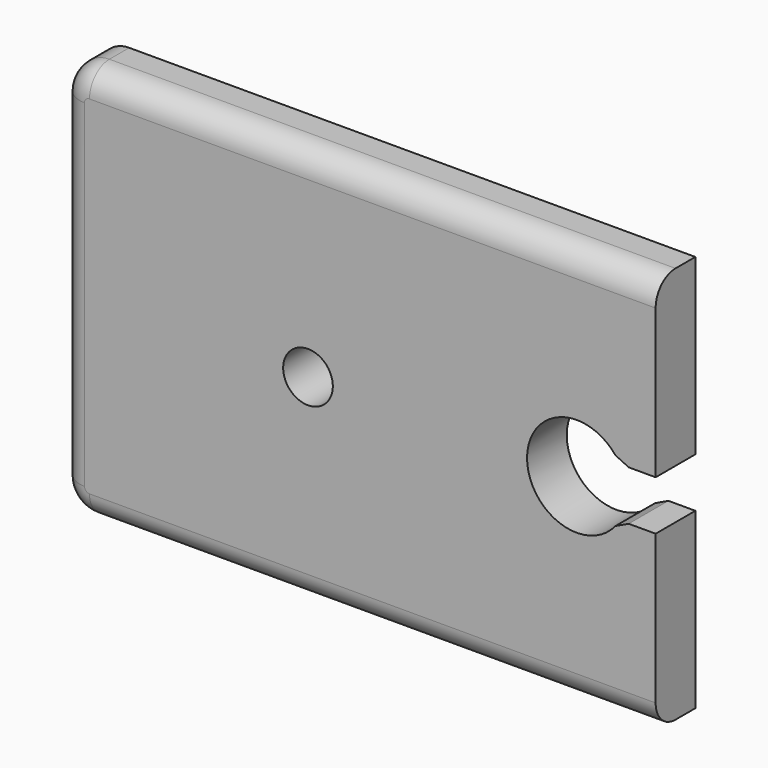
from build123d import *

# Parameters (mm, degrees)
F0_R        = 5
F1_DEPTH    = 10
F2_DEPTH    = 23.2
F3_R        = 6
F4_T1_DEPTH = 19.4160695157
F5_R        = 5


# Not quite as in the source:
# - a fillet or chamfer that OpenCascade refuses, or shapes differently, is made with other operations: its cross-section is extruded or revolved along the edge and cut away or added


with BuildPart() as f1:
    # F0 (on Front) → F1 (new body)
    with BuildSketch(Plane.XZ):
        with BuildLine():
            Line((53.1680434942, 40), (-66.8319565058, 40))
            Line((-66.8319565058, 40), (-66.8319565058, -40))
            Line((-66.8319565058, -40), (53.1680434942, -40))
            Line((53.1680434942, -40), (53.1680434942, -5))
            Line((53.1680434942, -5), (47.2735762596, -5))
            Line((47.2735762596, -5), (45.9338302975, -5))
            ThreePointArc((45.9338302975, -5), (27.2735762596, 0), (45.9338302975, 5))
            Line((45.9338302975, 5), (47.2735762596, 5))
            Line((47.2735762596, 5), (53.1680434942, 5))
            Line((53.1680434942, 5), (53.1680434942, 40))
        make_face()
        with Locations((-16.8319565058, 0)):
            Circle(F0_R, mode=Mode.SUBTRACT)
    extrude(amount=F1_DEPTH)

    # F0 (on Front) → F2 (cut)
    with BuildSketch(Plane.XZ):
        with Locations((-16.8319565058, 0)):
            Circle(F0_R)
    extrude(amount=-F2_DEPTH, mode=Mode.SUBTRACT)

    # F3
    f3_edges = [f1.edges().sort_by_distance(p)[0] for p in [
        (-66.831957, -5, -40),
        (-66.831957, -5, 40),
    ]]
    fillet(f3_edges, radius=F3_R)

    # F4: chamfer of 2 on 2 edges, made by hand

    # F4_s2 → F4_t1 (cut)
    with BuildSketch(Plane.XZ.offset(-4.7080347579)):
        with BuildLine():
            Line((44.9783315762, -6.3208937548), (47.8167286643, -4.9655276174))
            Line((47.8167286643, -4.9655276174), (47.8167286643, -4.9255276174))
            ThreePointArc((47.8167286643, -4.9255276174), (46.8752794809, -4.96), (45.9338302975, -4.96))
            Line((45.9338302975, -4.96), (45.8991892813, -4.98))
            ThreePointArc((45.8991892813, -4.98), (45.4646544727, -5.6663778296), (44.9472237878, -6.2957480693))
            Line((44.9472237878, -6.2957480693), (44.9783315762, -6.3208937548))
        make_face()
        with BuildLine():
            Line((47.8167286643, 4.9655276174), (44.9783315762, 6.3208937548))
            Line((44.9783315762, 6.3208937548), (44.9472237878, 6.2957480693))
            ThreePointArc((44.9472237878, 6.2957480693), (45.4646544727, 5.6663778296), (45.8991892813, 4.98))
            Line((45.8991892813, 4.98), (45.9338302975, 4.96))
            ThreePointArc((45.9338302975, 4.96), (46.8752794809, 4.96), (47.8167286643, 4.9255276174))
            Line((47.8167286643, 4.9255276174), (47.8167286643, 4.9655276174))
        make_face()
    extrude(amount=F4_T1_DEPTH, mode=Mode.SUBTRACT)

    # F5
    f5_edges = [f1.edges().sort_by_distance(p)[0] for p in [
        (-3.831957, -10, -40),
        (-3.831957, -10, 40),
        (-65.074597, -10, 38.242641),
        (-65.074597, -10, -38.242641),
        (-66.831957, -10, 0),
    ]]
    fillet(f5_edges, radius=F5_R)


solid = f1.part
